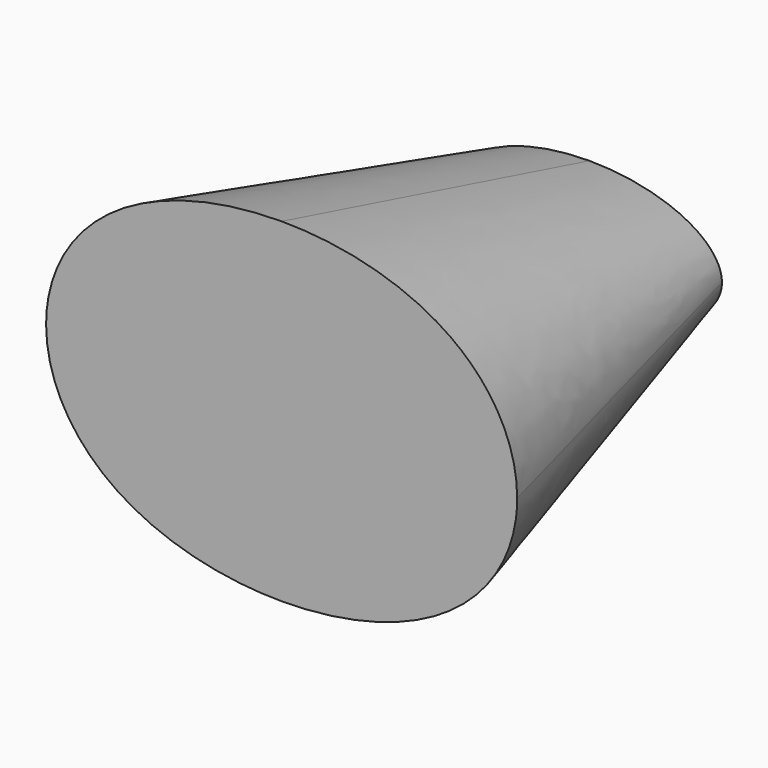
from build123d import *

# Parameters (mm, degrees)
F1_DEPTH = 381
F1_TAPER = -15


with BuildPart() as f1:
    # F0 (on Front) → F1 (new body)
    with BuildSketch(Plane.XZ):
        with BuildLine():
            add(Edge.make_bspline(
                [(131.1613061313, 13.49375), (131.1613061313, 123.4789762806), (-65.5806530657, 68.4863631403), (-262.3226122627, 13.49375), (-65.5806530657, -41.4988631403), (131.1613061313, -96.4914762806), (131.1613061313, 13.49375)],
                knots=[0, 0, 0, 2.0943951024, 2.0943951024, 4.1887902048, 4.1887902048, 6.2831853072, 6.2831853072, 6.2831853072], degree=2, weights=[1, 0.5, 1, 0.5, 1, 0.5, 1]))
        make_face()
    extrude(amount=F1_DEPTH, taper=F1_TAPER)


solid = f1.part
